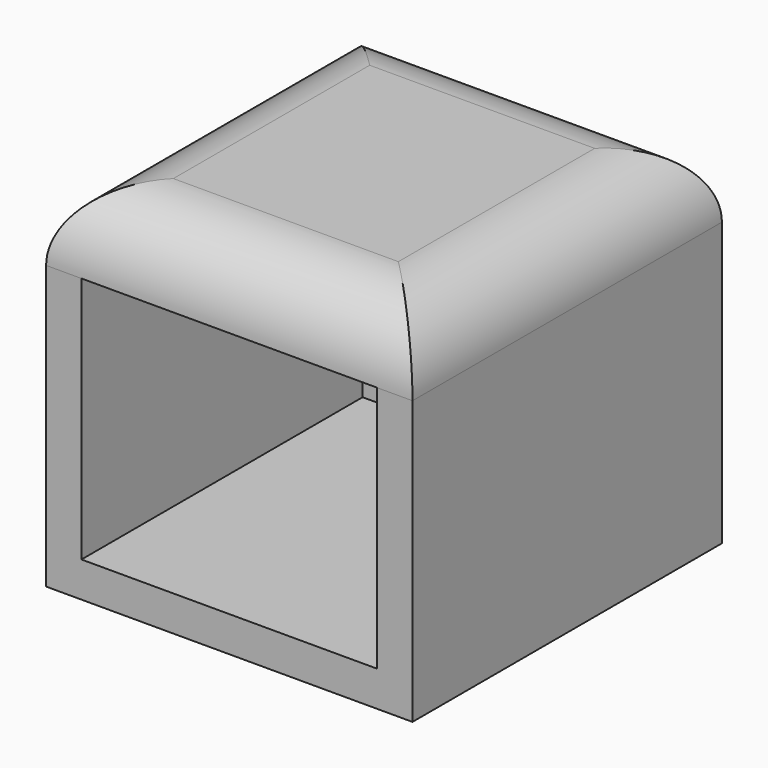
from build123d import *

# Parameters (mm, degrees)
F0_W     = 26.3287108392
F0_H     = 27.7948193252
F1_DEPTH = 25.4
F2_R     = 5.08
F3_T     = -2.54


# Not quite as in the source:
# - a shell that OpenCascade refuses in one call is made with other operations: the cavity is built on its own and cut out


with BuildPart() as f1:
    # F0 (on Top) → F1 (new body)
    with BuildSketch(Plane.XY):
        with Locations((-13.1643554196, 13.1417736411)):
            Rectangle(F0_W, F0_H)
    extrude(amount=F1_DEPTH)

    # F2
    f2_edges = [f1.edges().sort_by_distance(p)[0] for p in [
        (-26.328711, 13.141774, 25.4),
        (-13.164355, -0.755636, 25.4),
        (0, 13.141774, 25.4),
        (-13.164355, 27.039183, 25.4),
    ]]
    fillet(f2_edges, radius=F2_R)

    # F3: a shell. OpenCascade refuses it in one call, so the cavity is built on its own and cut out:
    # the body offset inwards by the wall thickness, plus a prism from it out through each open face.
    f3_core = offset(f1.part, amount=F3_T, mode=Mode.PRIVATE)
    f3_exits = [f3_core.faces().sort_by_distance(p)[0] for p in [
        (-13.164355, 1.784364, 11.43),
    ]]
    add(f3_core, mode=Mode.SUBTRACT)
    extrude(f3_exits, amount=-F3_T, mode=Mode.SUBTRACT)


solid = f1.part
